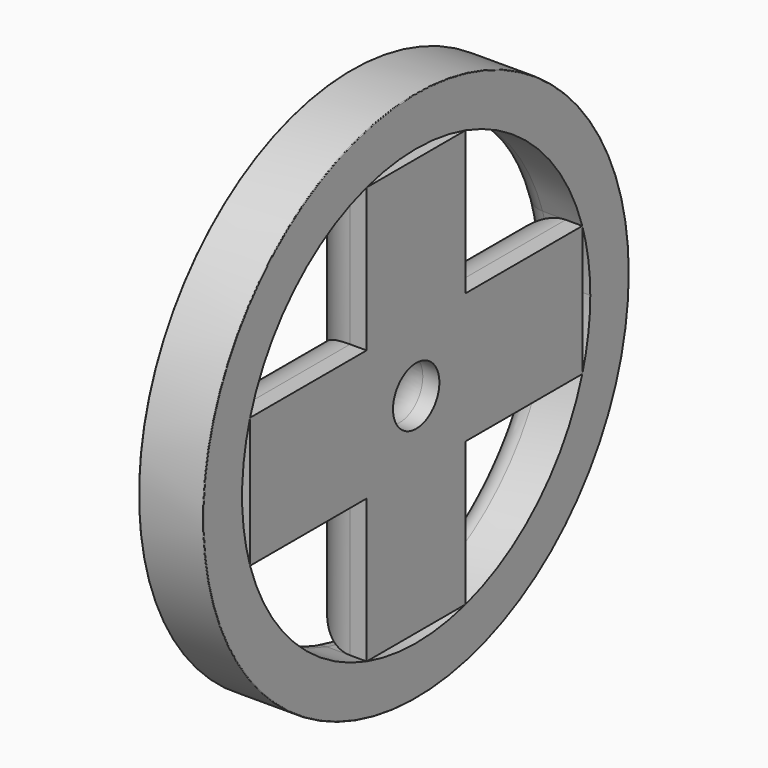
from build123d import *

# Parameters (mm, degrees)
F0_R         = 10.3021745403
F1_DEPTH     = 2.5
F0_R_2       = 1.1222237914
F3_DEPTH     = 2.5
F4_T1_DEPTH  = 10.2881459995
F4_T3_DEPTH  = 14.3412472678
F4_T5_DEPTH  = 10.2011818375
F4_T7_DEPTH  = 14.0908572342
F4_T9_DEPTH  = 10.2881459995
F4_T11_DEPTH = 10.2011818375
F4_T19_DEPTH = 14.9355071071
F4_T23_DEPTH = 14.8485429451
F4_T30_DEPTH = 14.9355071071
F4_T34_DEPTH = 14.8485429451
F4_T41_DEPTH = 14.8485429451
F4_T45_DEPTH = 14.9355071071
F4_T52_DEPTH = 14.9355071071
F4_T56_DEPTH = 14.8485429451
F5_R         = 0.9656854249
F6_R         = 0.0241421356


# Not quite as in the source:
# - a fillet or chamfer that OpenCascade refuses, or shapes differently, is made with other operations: its cross-section is extruded or revolved along the edge and cut away or added
# - a feature of the source that left no trace in its solid (it failed there, or was rolled back) is left out


with BuildPart() as f1:
    # F0 (on Right) → F1 (new body)
    with BuildSketch(Plane.YZ):
        Circle(F0_R)
        with BuildLine():
            ThreePointArc((8.0388524015, 2.5232625263), (8.3283193537, 1.2763614112), (8.4255564629, 0))
            ThreePointArc((8.4255564629, 0), (8.3283193537, -1.2763614112), (8.0388524015, -2.5232625263))
            ThreePointArc((8.0388524015, -2.5232625263), (5.9113074258, -6.0038692713), (2.3980675096, -8.0770832563))
            ThreePointArc((2.3980675096, -8.0770832563), (0, -8.4255564629), (-2.3980675096, -8.0770832563))
            ThreePointArc((-2.3980675096, -8.0770832563), (-5.9113074258, -6.0038692713), (-8.0388524015, -2.5232625263))
            ThreePointArc((-8.0388524015, -2.5232625263), (-8.4255564629, 0), (-8.0388524015, 2.5232625263))
            ThreePointArc((-8.0388524015, 2.5232625263), (-5.9113074258, 6.0038692713), (-2.3980675096, 8.0770832563))
            ThreePointArc((-2.3980675096, 8.0770832563), (0, 8.4255564629), (2.3980675096, 8.0770832563))
            ThreePointArc((2.3980675096, 8.0770832563), (5.9113074258, 6.0038692713), (8.0388524015, 2.5232625263))
        make_face(mode=Mode.SUBTRACT)
    extrude(amount=F1_DEPTH)

    # F5
    f5_edges = [f1.edges().sort_by_distance(p)[0] for p in [
        (0, 8.038852, 2.523263),
    ]]
    fillet(f5_edges, radius=F5_R)

    # F6
    f6_edges = [f1.edges().sort_by_distance(p)[0] for p in [
        (1.25, 10.302175, 0),
        (0, -10.302175, 0),
        (2.5, -10.302175, 0),
    ]]
    fillet(f6_edges, radius=F6_R)


with BuildPart() as f3:
    # F0 (on Right) → F3 (new body)
    with BuildSketch(Plane.YZ):
        Polygon((8.0388524015, -2.5232625263), (8.0388524015, 2.5232625263), (2.3980675096, 2.5232625263), (2.3980675096, 8.0770832563), (-2.3980675096, 8.0770832563), (-2.3980675096, 2.5232625263), (-8.0388524015, 2.5232625263), (-8.0388524015, -2.5232625263), (-2.3980675096, -2.5232625263), (-2.3980675096, -8.0770832563), (2.3980675096, -8.0770832563), (2.3980675096, -2.5232625263), align=None)
        Circle(F0_R_2, mode=Mode.SUBTRACT)
    extrude(amount=F3_DEPTH)

    # F4: fillet of radius 1.858944443 on 13 edges, made by hand

    # F4_s2 → F4_t1 (cut)
    with BuildSketch(Plane.XZ.offset(-12.686213509)):
        with BuildLine():
            ThreePointArc((1.858944443, -2.5232625263), (0.5444722215, -1.9787903048), (0, -0.6643180833))
            Line((0, -0.6643180833), (0, -2.5232625263))
            Line((0, -2.5232625263), (1.858944443, -2.5232625263))
        make_face()
        with BuildLine():
            ThreePointArc((1.858944443, 2.5232625263), (0.5444722215, 1.9787903048), (0, 0.6643180833))
            Line((0, 0.6643180833), (0, 2.5232625263))
            Line((0, 2.5232625263), (1.858944443, 2.5232625263))
        make_face()
    extrude(amount=F4_T1_DEPTH, mode=Mode.SUBTRACT)

    # F4_s4 → F4_t3 (cut)
    with BuildSketch(Plane.XY.offset(-7.1706236339)):
        with BuildLine():
            ThreePointArc((1.858944443, 8.0388524015), (0.5444722215, 7.49438018), (0, 6.1799079584))
            Line((0, 6.1799079584), (0, 8.0388524015))
            Line((0, 8.0388524015), (1.858944443, 8.0388524015))
        make_face()
        with BuildLine():
            ThreePointArc((1.858944443, -8.0388524015), (0.5444722215, -7.49438018), (0, -6.1799079584))
            Line((0, -6.1799079584), (0, -8.0388524015))
            Line((0, -8.0388524015), (1.858944443, -8.0388524015))
        make_face()
    extrude(amount=F4_T3_DEPTH, mode=Mode.SUBTRACT)

    # F4_s6 → F4_t5 (cut)
    with BuildSketch(Plane.XY.offset(2.5232625263)):
        with BuildLine():
            ThreePointArc((1.858944443, 2.3980675096), (0.5444722215, 1.853595288), (0, 0.5391230665))
            Line((0, 0.5391230665), (0, 2.3980675096))
            Line((0, 2.3980675096), (1.858944443, 2.3980675096))
        make_face()
        with BuildLine():
            ThreePointArc((1.858944443, -2.3980675096), (0.5444722215, -1.853595288), (0, -0.5391230665))
            Line((0, -0.5391230665), (0, -2.3980675096))
            Line((0, -2.3980675096), (1.858944443, -2.3980675096))
        make_face()
    extrude(amount=F4_T5_DEPTH, mode=Mode.SUBTRACT)

    # F4_s8 → F4_t7 (cut)
    with BuildSketch(Plane.XZ.offset(-7.0454286171)):
        with BuildLine():
            ThreePointArc((1.858944443, 8.0770832563), (0.5444722215, 7.5326110348), (0, 6.2181388133))
            Line((0, 6.2181388133), (0, 8.0770832563))
            Line((0, 8.0770832563), (1.858944443, 8.0770832563))
        make_face()
        with BuildLine():
            ThreePointArc((1.858944443, -8.0770832563), (0.5444722215, -7.5326110348), (0, -6.2181388133))
            Line((0, -6.2181388133), (0, -8.0770832563))
            Line((0, -8.0770832563), (1.858944443, -8.0770832563))
        make_face()
    extrude(amount=F4_T7_DEPTH, mode=Mode.SUBTRACT)

    # F4_s10 → F4_t9 (cut)
    with BuildSketch(Plane.XZ.offset(2.3980675096)):
        with BuildLine():
            ThreePointArc((1.858944443, 2.5232625263), (0.5444722215, 1.9787903048), (0, 0.6643180833))
            Line((0, 0.6643180833), (0, 2.5232625263))
            Line((0, 2.5232625263), (1.858944443, 2.5232625263))
        make_face()
        with BuildLine():
            ThreePointArc((1.858944443, -2.5232625263), (0.5444722215, -1.9787903048), (0, -0.6643180833))
            Line((0, -0.6643180833), (0, -2.5232625263))
            Line((0, -2.5232625263), (1.858944443, -2.5232625263))
        make_face()
    extrude(amount=F4_T9_DEPTH, mode=Mode.SUBTRACT)

    # F4_s12 → F4_t11 (cut)
    with BuildSketch(Plane.XY.offset(-12.7244443639)):
        with BuildLine():
            ThreePointArc((1.858944443, -2.3980675096), (0.5444722215, -1.853595288), (0, -0.5391230665))
            Line((0, -0.5391230665), (0, -2.3980675096))
            Line((0, -2.3980675096), (1.858944443, -2.3980675096))
        make_face()
        with BuildLine():
            ThreePointArc((1.858944443, 2.3980675096), (0.5444722215, 1.853595288), (0, 0.5391230665))
            Line((0, 0.5391230665), (0, 2.3980675096))
            Line((0, 2.3980675096), (1.858944443, 2.3980675096))
        make_face()
    extrude(amount=F4_T11_DEPTH, mode=Mode.SUBTRACT)

    # F4_s13 → F4_t14 (revolve, cut)
    with BuildSketch(Plane.XY):
        with BuildLine():
            ThreePointArc((1.858944443, 1.1222237914), (0.5444722215, 1.666696013), (0, 2.9811682345))
            Line((0, 2.9811682345), (0, 1.1222237914))
            Line((0, 1.1222237914), (1.858944443, 1.1222237914))
        make_face()
    revolve(axis=Axis((0, 0, 0), (1, 0, 0)), mode=Mode.SUBTRACT)


with BuildPart() as f4_tool17:
    # F4_s18 → F4_t19 (new body)
    with BuildSketch(Plane.XZ.offset(2.249293598)):
        with BuildLine():
            ThreePointArc((1.858944443, -2.5232625263), (0.5444722215, -1.9787903048), (0, -0.6643180833))
            Line((0, -0.6643180833), (0, -2.5232625263))
            Line((0, -2.5232625263), (1.858944443, -2.5232625263))
        make_face()
    extrude(amount=-F4_T19_DEPTH)

    split(bisect_by=Plane.XZ.offset(-2.3980675096), keep=Keep.TOP)


with BuildPart() as f4_tool21:
    # F4_s22 → F4_t23 (new body)
    with BuildSketch(Plane.XY.offset(-12.7244443639)):
        with BuildLine():
            ThreePointArc((1.858944443, 2.3980675096), (0.5444722215, 1.853595288), (0, 0.5391230665))
            Line((0, 0.5391230665), (0, 2.3980675096))
            Line((0, 2.3980675096), (1.858944443, 2.3980675096))
        make_face()
    extrude(amount=F4_T23_DEPTH)

    split(bisect_by=Plane.XY.offset(-2.5232625263), keep=Keep.TOP)


with BuildPart() as f4_tool17_1:
    add(f4_tool17.part)

    # F4_t25: intersect F4_tool21
    add(f4_tool21.part, mode=Mode.INTERSECT)


with BuildPart() as f3_1:
    add(f3.part)

    # F4_t15: cut F4_tool17
    add(f4_tool17_1.part, mode=Mode.SUBTRACT)


with BuildPart() as f4_tool28:
    # F4_s29 → F4_t30 (new body)
    with BuildSketch(Plane.XZ.offset(-12.686213509)):
        with BuildLine():
            ThreePointArc((1.858944443, 2.5232625263), (0.5444722215, 1.9787903048), (0, 0.6643180833))
            Line((0, 0.6643180833), (0, 2.5232625263))
            Line((0, 2.5232625263), (1.858944443, 2.5232625263))
        make_face()
    extrude(amount=F4_T30_DEPTH)

    split(bisect_by=Plane.XZ.offset(-2.3980675096), keep=Keep.TOP)


with BuildPart() as f4_tool32:
    # F4_s33 → F4_t34 (new body)
    with BuildSketch(Plane.XY.offset(-2.1240985812)):
        with BuildLine():
            ThreePointArc((1.858944443, 2.3980675096), (0.5444722215, 1.853595288), (0, 0.5391230665))
            Line((0, 0.5391230665), (0, 2.3980675096))
            Line((0, 2.3980675096), (1.858944443, 2.3980675096))
        make_face()
    extrude(amount=F4_T34_DEPTH)

    split(bisect_by=Plane.XY.offset(2.5232625263), keep=Keep.BOTTOM)


with BuildPart() as f4_tool28_1:
    add(f4_tool28.part)

    # F4_t36: intersect F4_tool32
    add(f4_tool32.part, mode=Mode.INTERSECT)


with BuildPart() as f3_2:
    add(f3_1.part)

    # F4_t26: cut F4_tool28
    add(f4_tool28_1.part, mode=Mode.SUBTRACT)


with BuildPart() as f4_tool39:
    # F4_s40 → F4_t41 (new body)
    with BuildSketch(Plane.XY.offset(12.7244443639)):
        with BuildLine():
            ThreePointArc((1.858944443, -2.3980675096), (0.5444722215, -1.853595288), (0, -0.5391230665))
            Line((0, -0.5391230665), (0, -2.3980675096))
            Line((0, -2.3980675096), (1.858944443, -2.3980675096))
        make_face()
    extrude(amount=-F4_T41_DEPTH)

    split(bisect_by=Plane.XY.offset(2.5232625263), keep=Keep.BOTTOM)


with BuildPart() as f4_tool43:
    # F4_s44 → F4_t45 (new body)
    with BuildSketch(Plane.XZ.offset(-2.249293598)):
        with BuildLine():
            ThreePointArc((1.858944443, 2.5232625263), (0.5444722215, 1.9787903048), (0, 0.6643180833))
            Line((0, 0.6643180833), (0, 2.5232625263))
            Line((0, 2.5232625263), (1.858944443, 2.5232625263))
        make_face()
    extrude(amount=F4_T45_DEPTH)

    split(bisect_by=Plane.XZ.offset(2.3980675096), keep=Keep.BOTTOM)


with BuildPart() as f4_tool39_1:
    add(f4_tool39.part)

    # F4_t47: intersect F4_tool43
    add(f4_tool43.part, mode=Mode.INTERSECT)


with BuildPart() as f3_3:
    add(f3_2.part)

    # F4_t37: cut F4_tool39
    add(f4_tool39_1.part, mode=Mode.SUBTRACT)


with BuildPart() as f4_tool50:
    # F4_s51 → F4_t52 (new body)
    with BuildSketch(Plane.XZ.offset(12.686213509)):
        with BuildLine():
            ThreePointArc((1.858944443, -2.5232625263), (0.5444722215, -1.9787903048), (0, -0.6643180833))
            Line((0, -0.6643180833), (0, -2.5232625263))
            Line((0, -2.5232625263), (1.858944443, -2.5232625263))
        make_face()
    extrude(amount=-F4_T52_DEPTH)

    split(bisect_by=Plane.XZ.offset(2.3980675096), keep=Keep.BOTTOM)


with BuildPart() as f4_tool54:
    # F4_s55 → F4_t56 (new body)
    with BuildSketch(Plane.XY.offset(2.1240985812)):
        with BuildLine():
            ThreePointArc((1.858944443, -2.3980675096), (0.5444722215, -1.853595288), (0, -0.5391230665))
            Line((0, -0.5391230665), (0, -2.3980675096))
            Line((0, -2.3980675096), (1.858944443, -2.3980675096))
        make_face()
    extrude(amount=-F4_T56_DEPTH)

    split(bisect_by=Plane.XY.offset(-2.5232625263), keep=Keep.TOP)


with BuildPart() as f4_tool50_1:
    add(f4_tool50.part)

    # F4_t58: intersect F4_tool54
    add(f4_tool54.part, mode=Mode.INTERSECT)


with BuildPart() as f3_4:
    add(f3_3.part)

    # F4_t48: cut F4_tool50
    add(f4_tool50_1.part, mode=Mode.SUBTRACT)


solid = Compound([f1.part, f3_4.part])
